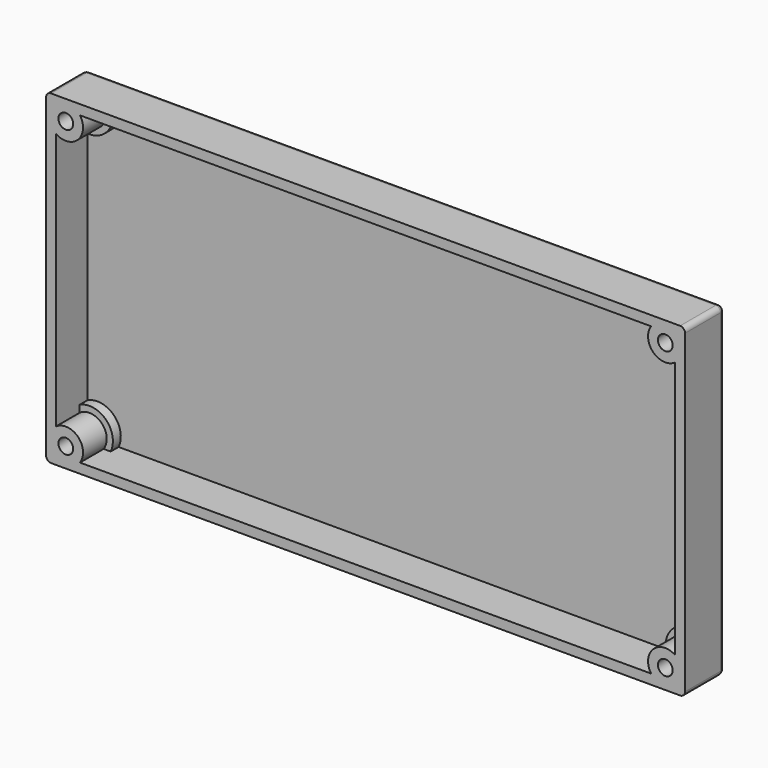
from build123d import *

# Parameters (mm, degrees)
F0_W           = 129.58
F0_H           = 66
F1_DEPTH       = 10
F3_D           = 3
F3_DEPTH       = 11
F3_CBORE_D     = 5.5
F3_CBORE_DEPTH = 2
F3_TIP         = 0.9012909285
F4_T           = 2
F5_R           = 1


# Not quite as in the source:
# - a shell that OpenCascade refuses in one call is made with other operations: the cavity is built on its own and cut out


with BuildPart() as f1:
    # F0 (on Front) → F1 (new body)
    with BuildSketch(Plane.XZ):
        with Locations((64.79, 33)):
            Rectangle(F0_W, F0_H)
    extrude(amount=F1_DEPTH)

    # F3
    with Locations(Plane(origin=(0, 0, 0), x_dir=(1, 0, 0), z_dir=(0, 1, 0))):
        with Locations((4, -62), (4, -4), (125.58, -4), (125.58, -62)):
            CounterBoreHole(F3_D / 2, F3_CBORE_D / 2, F3_CBORE_DEPTH, depth=F3_DEPTH)
            with Locations((0, 0, -(F3_DEPTH + F3_TIP / 2))):  # 118° drill point
                Cone(0, F3_D / 2, F3_TIP, mode=Mode.SUBTRACT)

    # F4: shell of thickness 2, made by hand


with BuildPart() as f4_core1:
    # F4_t2: copy of F1
    add(f1.part)

    # the walls: a layer under each face that stays
    f4_faces = [f4_core1.faces().sort_by_distance(p)[0] for p in [
        (0, -5, 33),
        (64.79, -5, 66),
        (64.79, -5, 0),
        (64.79, 0, 33),
        (129.58, -5, 33),
        (1.25, -1, 4),
        (122.83, -1, 4),
        (1.25, -1, 62),
        (122.83, -1, 62),
        (2.5, -6, 4),
        (124.08, -6, 4),
        (2.5, -6, 62),
        (124.08, -6, 62),
        (2.1666666667, -2, 5.8333333333),
        (123.7466666667, -2, 5.8333333333),
        (2.1666666667, -2, 63.8333333333),
        (123.7466666667, -2, 63.8333333333),
    ]]
    thicken(f4_faces, amount=-F4_T, mode=Mode.SUBTRACT)

    # F4_s3 → F4_t4 (revolve, cut)
    with BuildSketch(Plane.XY.offset(4)):
        Polygon((6.73, -1.98), (8.75, -2), (8.75, -4), (6.75, -4), align=None)
    revolve(axis=Axis((4, -2, 4), (0, 1, 0)), mode=Mode.SUBTRACT)

    # F4_s5 → F4_t6 (revolve, cut)
    with BuildSketch(Plane.XY.offset(4)):
        Polygon((128.31, -1.98), (130.33, -2), (130.33, -4), (128.33, -4), align=None)
    revolve(axis=Axis((125.58, -2, 4), (0, 1, 0)), mode=Mode.SUBTRACT)

    # F4_s7 → F4_t8 (revolve, cut)
    with BuildSketch(Plane.XY.offset(62)):
        Polygon((6.73, -1.98), (8.75, -2), (8.75, -4), (6.75, -4), align=None)
    revolve(axis=Axis((4, -2, 62), (0, 1, 0)), mode=Mode.SUBTRACT)

    # F4_s9 → F4_t10 (revolve, cut)
    with BuildSketch(Plane.XY.offset(62)):
        Polygon((128.31, -1.98), (130.33, -2), (130.33, -4), (128.33, -4), align=None)
    revolve(axis=Axis((125.58, -2, 62), (0, 1, 0)), mode=Mode.SUBTRACT)


with BuildPart() as f1_1:
    add(f1.part)

    # what is left inside the walls is the cavity
    f4_cavity = [f4_core1.part.solids().sort_by_distance(p)[0] for p in [
        (64.79, -9.98, 22.666667),
    ]]
    add(f4_cavity, mode=Mode.SUBTRACT)

    # F5
    f5_edges = [f1_1.edges().sort_by_distance(p)[0] for p in [
        (129.58, 0, 33),
        (64.79, 0, 66),
        (0, 0, 33),
        (64.79, 0, 0),
        (129.58, -5, 66),
        (129.58, -5, 0),
        (0, -5, 0),
        (0, -5, 66),
    ]]
    fillet(f5_edges, radius=F5_R)


solid = f1_1.part
